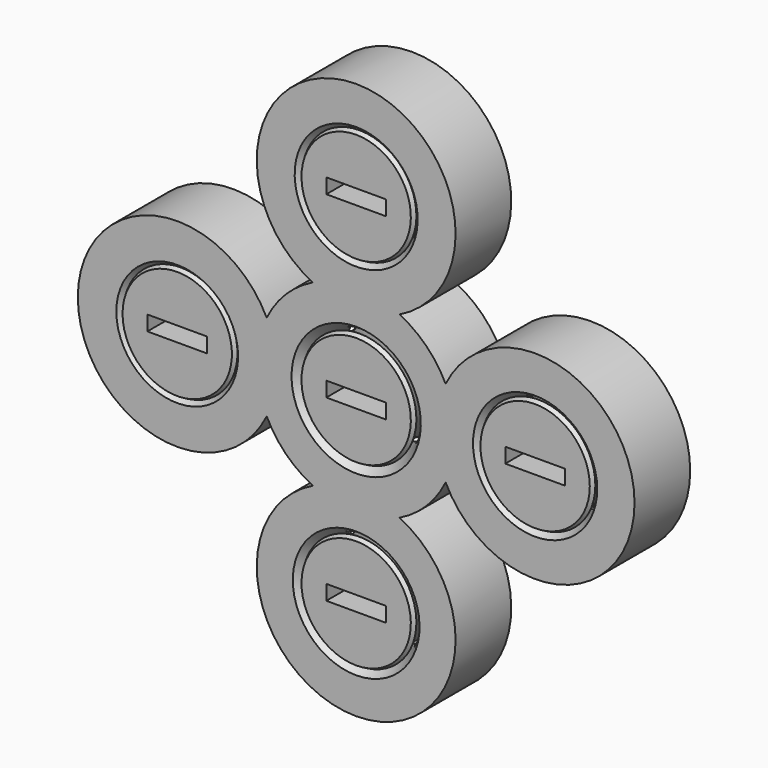
from build123d import *

# Parameters (mm, degrees)
F11_TEXT_SIZE   = 7.1408489021
F11_TEXT_SIZE_2 = 6.7808768815
F11_TEXT_SIZE_3 = 7.0120424627
F11_TEXT_SIZE_4 = 6.8683332453
F11_TEXT_SIZE_5 = 7.3867005995
F12_DEPTH       = 0.6
F13_W           = 6
F13_H           = 1.5
F14_DEPTH       = 4


# Not quite as in the source:
# - Text() gives the source's letters only with a copy of the font that has no kerning and outlines rounded to 1/6400 em; it was checked with that copy


with BuildPart() as f1:
    # F0 (on Top) → F1 (revolve)
    with BuildSketch(Plane.XY):
        with BuildLine():
            Line((-23.7255081441, 0.417916524), (-23.5, 0))
            Line((-23.5, 0), (-18, 0))
            Line((-18, 0), (-18, 7))
            Line((-18, 7), (-23.5, 7))
            Line((-23.5, 7), (-23.7255081441, 6.582083476))
            ThreePointArc((-23.7255081441, 6.582083476), (-22.8733971724, 3.5), (-23.7255081441, 0.417916524))
        make_face()
    revolve(axis=Axis((-18, 3.5, 0), (0, 1, 0)))


with BuildPart() as f1b:
    # F0 (on Top) → F1, piece 2 (revolve)
    with BuildSketch(Plane.XY):
        with BuildLine():
            Line((-28, 0), (-24.1236603376, 0))
            ThreePointArc((-24.1236603376, 0), (-22.9733971724, 3.5), (-24.1236603376, 7))
            Line((-24.1236603376, 7), (-28, 7))
            Line((-28, 7), (-28, 0))
        make_face()
    revolve(axis=Axis((-18, 3.5, 0), (0, 1, 0)))



with BuildPart() as f3:
    # F2 (on Right) → F3 (revolve)
    with BuildSketch(Plane.YZ):
        with BuildLine():
            Line((0.417916524, 23.7255081441), (0, 23.5))
            Line((0, 23.5), (0, 18))
            Line((0, 18), (7, 18))
            Line((7, 18), (7, 23.5))
            Line((7, 23.5), (6.582083476, 23.7255081441))
            ThreePointArc((6.582083476, 23.7255081441), (3.5, 22.8733971724), (0.417916524, 23.7255081441))
        make_face()
    revolve(axis=Axis((0, 3.5, 18), (0, 1, 0)))


with BuildPart() as f3b:
    # F2 (on Right) → F3, piece 2 (revolve)
    with BuildSketch(Plane.YZ):
        with BuildLine():
            Line((0, 28), (0, 24.1859138391))
            ThreePointArc((0, 24.1859138391), (3.5, 23.0233971724), (7, 24.1859138391))
            Line((7, 24.1859138391), (7, 28))
            Line((7, 28), (0, 28))
        make_face()
    revolve(axis=Axis((0, 3.5, 18), (0, 1, 0)))


with BuildPart() as f5:
    # F4 (on Top) → F5 (revolve)
    with BuildSketch(Plane.XY):
        with BuildLine():
            Line((23.7255081441, 6.582083476), (23.5, 7))
            Line((23.5, 7), (18, 7))
            Line((18, 7), (18, 0))
            Line((18, 0), (23.5, 0))
            Line((23.5, 0), (23.7257496965, 0.4175131041))
            ThreePointArc((23.7257496965, 0.4175131041), (22.873397177, 3.4997648962), (23.7255081441, 6.582083476))
        make_face()
    revolve(axis=Axis((18, 3.5, 0), (0, -1, 0)))


with BuildPart() as f5b:
    # F4 (on Top) → F5, piece 2 (revolve)
    with BuildSketch(Plane.XY):
        with BuildLine():
            Line((28, 7), (24.2484647405, 7))
            ThreePointArc((24.2484647405, 7), (23.0733971724, 3.5), (24.2484647405, 0))
            Line((24.2484647405, 0), (28, 0))
            Line((28, 0), (28, 7))
        make_face()
    revolve(axis=Axis((18, 3.5, 0), (0, -1, 0)))


with BuildPart() as f7:
    # F6 (on Right) → F7 (revolve)
    with BuildSketch(Plane.YZ):
        with BuildLine():
            Line((6.582083476, -23.7255081441), (7, -23.5))
            Line((7, -23.5), (7, -18))
            Line((7, -18), (0, -18))
            Line((0, -18), (0, -23.5))
            Line((0, -23.5), (0.417916524, -23.7255081441))
            ThreePointArc((0.417916524, -23.7255081441), (3.5, -22.8733971724), (6.582083476, -23.7255081441))
        make_face()
    revolve(axis=Axis((0, 3.5, -18), (0, -1, 0)))


with BuildPart() as f7b:
    # F6 (on Right) → F7, piece 2 (revolve)
    with BuildSketch(Plane.YZ):
        with BuildLine():
            Line((7, -28), (7, -24.3745084207))
            ThreePointArc((7, -24.3745084207), (3.5, -23.1733971724), (0, -24.3745084207))
            Line((0, -24.3745084207), (0, -28))
            Line((0, -28), (7, -28))
        make_face()
    revolve(axis=Axis((0, 3.5, -18), (0, -1, 0)))


with BuildPart() as f10:
    # F9 (on offset) → F10 (revolve)
    with BuildSketch(Plane.YZ):
        with BuildLine():
            Line((0.417916524, 5.7255081441), (0, 5.5))
            Line((0, 5.5), (0, 0))
            Line((0, 0), (7, 0))
            Line((7, 0), (7, 5.5))
            Line((7, 5.5), (6.582083476, 5.7255081441))
            ThreePointArc((6.582083476, 5.7255081441), (3.5, 4.8733971724), (0.417916524, 5.7255081441))
        make_face()
    revolve(axis=Axis((0, 3.5, 0), (0, 1, 0)))


with BuildPart() as f1b_1:
    add(f1b.part)

    add(f3b.part)  # F10#2 merges F3b

    add(f5b.part)  # F10#2 merges F5b

    add(f7b.part)  # F10#2 merges F7b
    # F9 (on offset) → F10, piece 2 (revolve)
    with BuildSketch(Plane.YZ):
        with BuildLine():
            Line((0, 10), (0, 6.5018985735))
            ThreePointArc((0, 6.5018985735), (3.5, 5.2733971724), (7, 6.5018985735))
            Line((7, 6.5018985735), (7, 10))
            Line((7, 10), (0, 10))
        make_face()
    revolve(axis=Axis((0, 3.5, 0), (0, 1, 0)))


with BuildPart() as f12_tool:
    # F11 (on face) → F12 (new body)
    with BuildSketch(Plane(origin=(0, 7, 0), x_dir=(-1, 0, 0), z_dir=(0, 1, 0))):
        with Locations((13.2093122229, -2.5772975641)):
            Text('0.1', F11_TEXT_SIZE, font='Open Sans', font_style=FontStyle.BOLD, text_align=(TextAlign.LEFT, TextAlign.BOTTOM))
        with Locations((-5.0139813684, 15.597583726)):
            Text('.15', F11_TEXT_SIZE_2, font='Open Sans', font_style=FontStyle.BOLD, text_align=(TextAlign.LEFT, TextAlign.BOTTOM))
        with Locations((-23.1004254892, -2.5443423074)):
            Text('0.2', F11_TEXT_SIZE_3, font='Open Sans', font_style=FontStyle.BOLD, text_align=(TextAlign.LEFT, TextAlign.BOTTOM))
        with Locations((-4.7190152109, -20.7702443004)):
            Text('0.3', F11_TEXT_SIZE_4, font='Open Sans', font_style=FontStyle.BOLD, text_align=(TextAlign.LEFT, TextAlign.BOTTOM))
        with Locations((-5.3721549921, -2.668940695)):
            Text('0.4', F11_TEXT_SIZE_5, font='Open Sans', font_style=FontStyle.BOLD, text_align=(TextAlign.LEFT, TextAlign.BOTTOM))
    extrude(amount=-F12_DEPTH)


with BuildPart() as f1_1:
    add(f1.part)

    # F12: cut by f12_tool
    add(f12_tool.part, mode=Mode.SUBTRACT)


with BuildPart() as f3_1:
    add(f3.part)

    # F12: cut by f12_tool
    add(f12_tool.part, mode=Mode.SUBTRACT)


with BuildPart() as f5_1:
    add(f5.part)

    # F12: cut by f12_tool
    add(f12_tool.part, mode=Mode.SUBTRACT)


with BuildPart() as f7_1:
    add(f7.part)

    # F12: cut by f12_tool
    add(f12_tool.part, mode=Mode.SUBTRACT)


with BuildPart() as f10_1:
    add(f10.part)

    # F12: cut by f12_tool
    add(f12_tool.part, mode=Mode.SUBTRACT)


with BuildPart() as f14_tool:
    # F13 (on face) → F14 (new body)
    with BuildSketch(Plane.XZ):
        with Locations((-18, 0)):
            Rectangle(F13_W, F13_H)
        Rectangle(F13_W, F13_H)
        with Locations((0, 18)):
            Rectangle(F13_W, F13_H)
        with Locations((18, 0)):
            Rectangle(F13_W, F13_H)
        with Locations((0, -18)):
            Rectangle(F13_W, F13_H)
    extrude(amount=-F14_DEPTH)


with BuildPart() as f1_2:
    add(f1_1.part)

    # F14: cut by f14_tool
    add(f14_tool.part, mode=Mode.SUBTRACT)


with BuildPart() as f3_2:
    add(f3_1.part)

    # F14: cut by f14_tool
    add(f14_tool.part, mode=Mode.SUBTRACT)


with BuildPart() as f5_2:
    add(f5_1.part)

    # F14: cut by f14_tool
    add(f14_tool.part, mode=Mode.SUBTRACT)


with BuildPart() as f7_2:
    add(f7_1.part)

    # F14: cut by f14_tool
    add(f14_tool.part, mode=Mode.SUBTRACT)


with BuildPart() as f10_2:
    add(f10_1.part)

    # F14: cut by f14_tool
    add(f14_tool.part, mode=Mode.SUBTRACT)


solid = Compound([f1b_1.part, f1_2.part, f3_2.part, f5_2.part, f7_2.part, f10_2.part])
